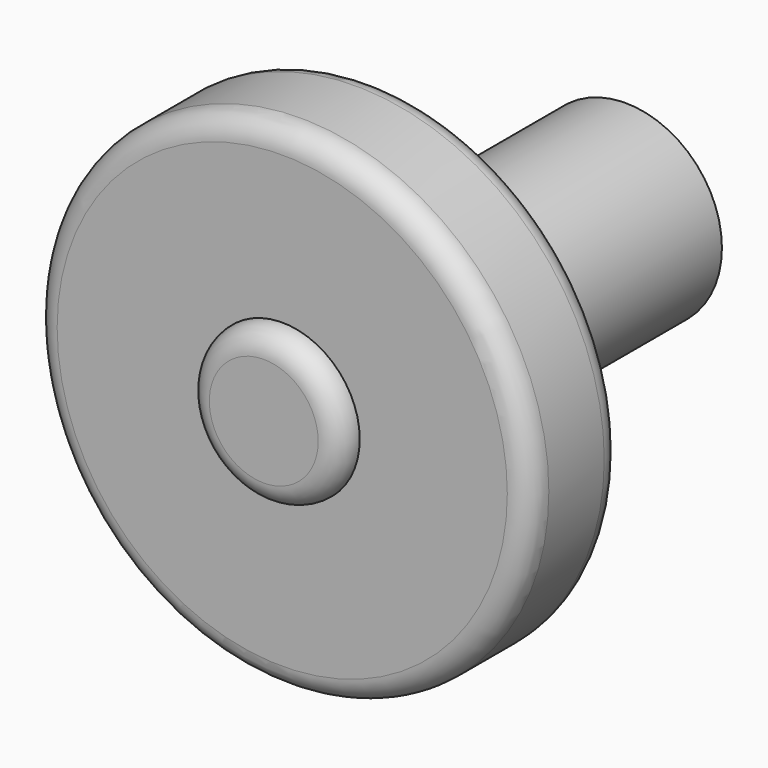
from build123d import *

# Parameters (mm, degrees)
F0_R      = 20.8649821503
F1_DEPTH  = 68
F2_R      = 53.7694879876
F2_R_2    = 20.8649821503
F3_DEPTH  = 25
F4_R      = 5.6100913923
F5_DEPTH  = 93.001
F7_R      = 5
F8_R      = 13.049224489
F8_R_2    = 5.6100913923
F9_DEPTH  = 10
F10_R     = 12.7052996832
F11_DEPTH = 5
F10_R_2   = 16.7944070529
F10_R_3   = 13.049224489
F12_DEPTH = 5
F13_R     = 4.99999


# Not quite as in the source:
# - a fillet or chamfer is up to 0.001 mm smaller than in the source, because OpenCascade refuses the exact size


with BuildPart() as f1:
    # F0 (on Front) → F1 (new body)
    with BuildSketch(Plane.XZ):
        Circle(F0_R)
    extrude(amount=F1_DEPTH)


with BuildPart() as f3:
    # F2 (on face) → F3 (new body)
    with BuildSketch(Plane.XZ.offset(68)):
        Circle(F2_R)
        Circle(F2_R_2, mode=Mode.SUBTRACT)
        Circle(F2_R_2)
    extrude(amount=F3_DEPTH)


with BuildPart() as f5:
    # F4 (on face) → F5 (new body, through all)
    with BuildSketch(Plane.XZ.offset(93)):
        Circle(F4_R)
    extrude(amount=-F5_DEPTH)


with BuildPart() as f1_1:
    add(f1.part)

    # F6: cut F5
    add(f5.part, mode=Mode.SUBTRACT)


with BuildPart() as f3_1:
    add(f3.part)

    # F6: cut F5
    add(f5.part, mode=Mode.SUBTRACT)

    # F7
    f7_edges = [f3_1.edges().sort_by_distance(p)[0] for p in [
        (-53.769488, -93, 0),
        (-53.769488, -68, 0),
    ]]
    fillet(f7_edges, radius=F7_R)

    # F8 (on face) → F9 (cut)
    with BuildSketch(Plane.XZ.offset(93)):
        Circle(F8_R)
        Circle(F8_R_2, mode=Mode.SUBTRACT)
    extrude(amount=-F9_DEPTH, mode=Mode.SUBTRACT)


with BuildPart() as f11:
    # F10 (on face) → F11 (new body)
    with BuildSketch(Plane.XZ.offset(93)):
        Circle(F10_R)
    extrude(amount=-F11_DEPTH)

    # F10 (on face) → F12 (join)
    with BuildSketch(Plane.XZ.offset(93)):
        Circle(F10_R_2)
        Circle(F10_R_3, mode=Mode.SUBTRACT)
        Circle(F10_R_3)
        Circle(F10_R, mode=Mode.SUBTRACT)
        Circle(F10_R)
    extrude(amount=F12_DEPTH)

    # F13 (radius 5 in the source; OpenCascade refuses exactly that, so slightly less here)
    f13_edges = [f11.edges().sort_by_distance(p)[0] for p in [
        (-16.794407, -98, 0),
    ]]
    fillet(f13_edges, radius=F13_R)


solid = Compound([f1_1.part, f3_1.part, f11.part])
